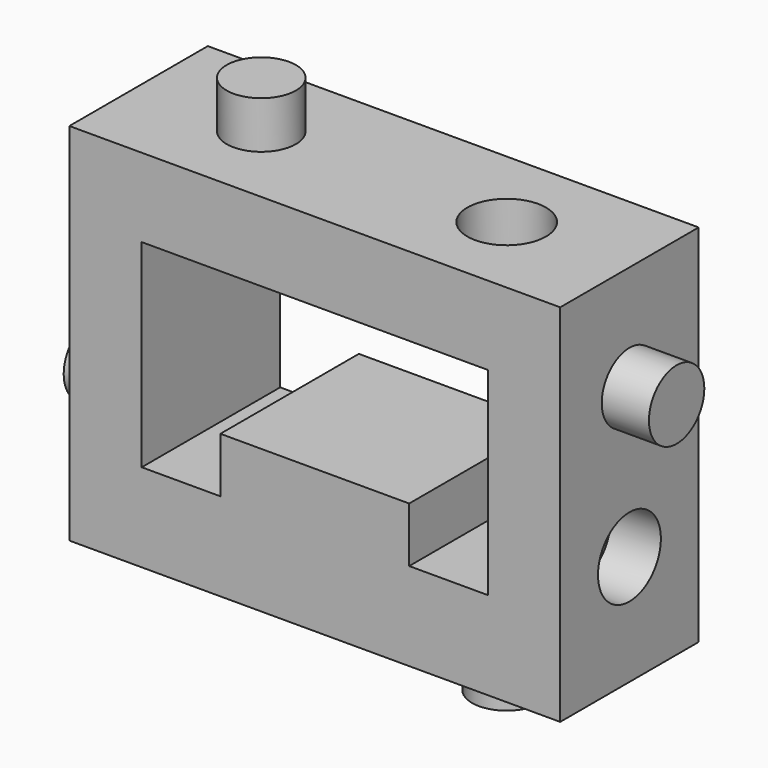
from build123d import *

# Parameters (mm, degrees)
F0_W      = 15.6
F0_H      = 11
F1_DEPTH  = 23.2
F3_DEPTH  = 25
F4_R      = 2.5
F5_DEPTH  = 3.2
F6_R      = 2.2
F7_DEPTH  = 3
F8_R      = 2.2
F9_DEPTH  = 3
F10_R     = 2.5
F11_DEPTH = 3
F13_R     = 2.2
F14_DEPTH = 3
F12_R     = 2.5
F15_DEPTH = 3.2
F16_R     = 2.5
F18_DEPTH = 3.2
F17_R     = 2.2
F19_DEPTH = 3


# Not quite as in the source:
# - a feature names something its author has since deleted; it is built from what else it names


with BuildPart() as f1:
    # F0 (on Top) → F1 (new body)
    with BuildSketch(Plane.XY):
        with Locations((-7.8, 0)):
            Rectangle(F0_W, F0_H)
        with Locations((7.8, 0)):
            Rectangle(F0_W, F0_H)
    extrude(amount=F1_DEPTH)

    # F2 (on face) → F3 (cut)
    with BuildSketch(Plane.XZ.offset(5.5)):
        Polygon((0, 18.2), (-11, 18.2), (-11, 5.6), (-6, 5.6), (-6, 9.1), (0, 9.1), (6, 9.1), (6, 5.6), (11, 5.6), (11, 18.2), align=None)
    extrude(amount=-F3_DEPTH, mode=Mode.SUBTRACT)

    # F4 (on face) → F5 (cut)
    with BuildSketch(Plane(origin=(0, 0, 0), x_dir=(1, 0, 0), z_dir=(0, 0, -1))):
        with Locations((-7.8, 0)):
            Circle(F4_R)
    extrude(amount=-F5_DEPTH, mode=Mode.SUBTRACT)

    # F6 (on face) → F7 (join)
    with BuildSketch(Plane(origin=(0, 0, 0), x_dir=(1, 0, 0), z_dir=(0, 0, -1))):
        with Locations((7.8, 0)):
            Circle(F6_R)
    extrude(amount=F7_DEPTH)

    # F8 (on face) → F9 (join)
    with BuildSketch(Plane.XY.offset(23.2)):
        with Locations((-7.8, 0)):
            Circle(F8_R)
    extrude(amount=F9_DEPTH)

    # F10 (on face) → F11 (cut)
    with BuildSketch(Plane.XY.offset(23.2)):
        with Locations((7.8, 0)):
            Circle(F10_R)
    extrude(amount=-F11_DEPTH, mode=Mode.SUBTRACT)

    # F13 (on face) → F14 (join)
    with BuildSketch(Plane.YZ.offset(15.6)):
        with Locations((0, 16.5)):
            Circle(F13_R)
    extrude(amount=F14_DEPTH)

    # F12 (on face) → F15 (cut)
    with BuildSketch(Plane.YZ.offset(15.6)):
        with Locations((0, 7)):
            Circle(F12_R)
    extrude(amount=-F15_DEPTH, mode=Mode.SUBTRACT)

    # F16 (on face) → F18 (cut)
    with BuildSketch(Plane(origin=(-15.6, 0, 0), x_dir=(0, -1, 0), z_dir=(-1, 0, 0))):
        with Locations((0, 16.5)):
            Circle(F16_R)
    extrude(amount=-F18_DEPTH, mode=Mode.SUBTRACT)

    # F17 (on face) → F19 (join)
    with BuildSketch(Plane(origin=(-15.6, 0, 0), x_dir=(0, -1, 0), z_dir=(-1, 0, 0))):
        with Locations((0, 7)):
            Circle(F17_R)
    extrude(amount=F19_DEPTH)


solid = f1.part
